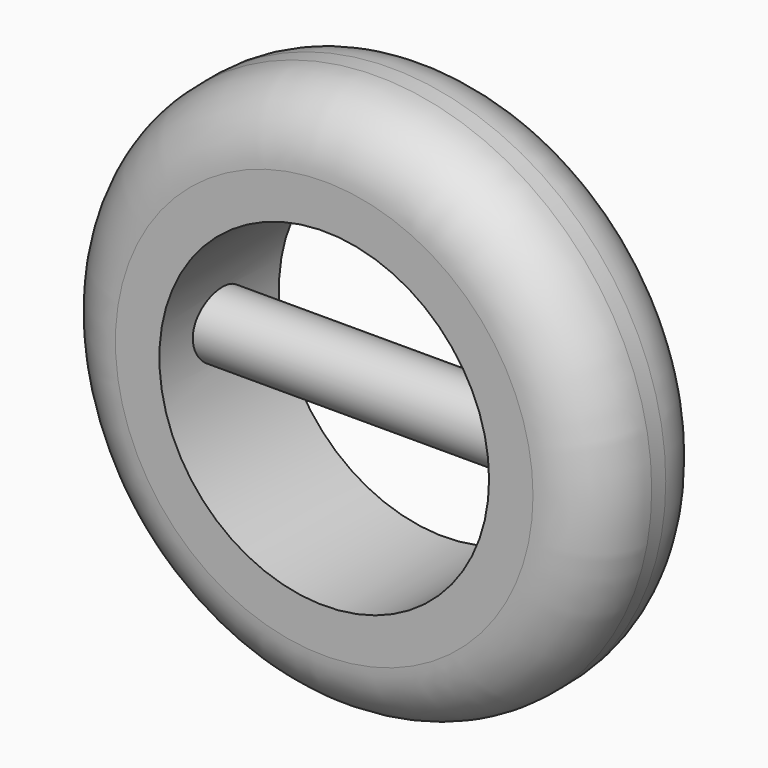
from build123d import *

# Parameters (mm, degrees)
F0_R     = 12.5
F0_R_2   = 7.5
F1_DEPTH = 3.4
F2_R     = 3
F4_R     = 1.5
F5_DEPTH = 10


# Not quite as in the source:
# - the program builds the solid bodies; features that only make, move or delete a surface that nothing else refers to are left out


with BuildPart() as f1:
    # F0 (on Front) → F1 (new body, symmetric)
    with BuildSketch(Plane.XZ):
        Circle(F0_R)
        Circle(F0_R_2, mode=Mode.SUBTRACT)
    extrude(amount=F1_DEPTH, both=True)

    # F2
    f2_edges = [f1.edges().sort_by_distance(p)[0] for p in [
        (-12.5, 3.4, 0),
        (-12.5, -3.4, 0),
    ]]
    fillet(f2_edges, radius=F2_R)

    # F4 (on Right) → F5 (join, symmetric)
    with BuildSketch(Plane.YZ):
        Circle(F4_R)
    extrude(amount=F5_DEPTH, both=True)


solid = f1.part
